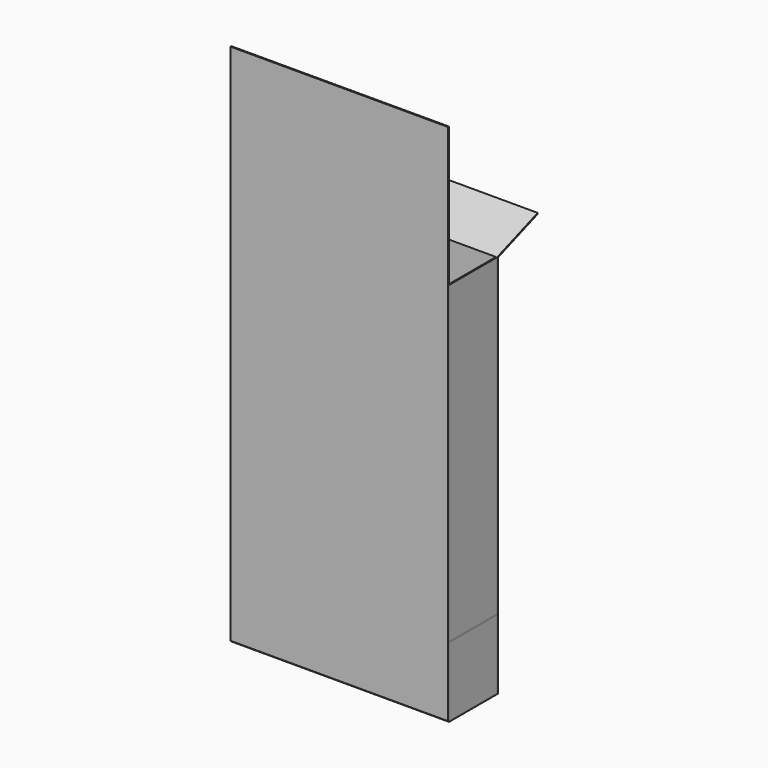
from build123d import *

# Parameters (mm, degrees)
F0_W      = 317.5
F0_H      = 762
F1_DEPTH  = 1.5875
F2_W      = 317.5
F2_H      = 88.9
F3_DEPTH  = 1.5875
F4_W      = 317.5
F4_H      = 558.8
F5_DEPTH  = 1.5875
F7_DEPTH  = 317.5
F8_DEPTH  = 1.5875
F11_DEPTH = 1.5875
F12_W     = 31.75
F12_H     = 78.7464009495
F13_DEPTH = 1.5875
F15_DEPTH = 2.54
F16_DEPTH = 1.5875
F6_W      = 87.3125
F6_H      = 1.5875
F17_DEPTH = 317.5
F6_H_2    = 100.0125
F18_DEPTH = 1.5875


# Not quite as in the source:
# - a length typed as a fraction of an inch, garbled in the dataset ("3 / 203.2 mm" for 3/8 in), is restored


with BuildPart() as f1:
    # F0 (on Front) → F1 (new body)
    with BuildSketch(Plane.XZ):
        Rectangle(F0_W, F0_H)
    extrude(amount=F1_DEPTH)


with BuildPart() as f3:
    # F2 (on face) → F3 (new body)
    with BuildSketch(Plane(origin=(0, 0, -381), x_dir=(1, 0, 0), z_dir=(0, 0, -1))):
        with Locations((0, -44.45)):
            Rectangle(F2_W, F2_H)
    extrude(amount=F3_DEPTH)

    # F4 (on face) → F5 (join)
    with BuildSketch(Plane(origin=(0, 88.9, 0), x_dir=(-1, 0, 0), z_dir=(0, 1, 0))):
        with Locations((0, -101.6)):
            Rectangle(F4_W, F4_H)
    extrude(amount=-F5_DEPTH)

    # F6 (on face) → F7 (join)
    with BuildSketch(Plane.YZ.offset(158.75)):
        Polygon((161.29, 204.7875), (87.3125, 177.8), (88.9, 177.8), (88.9, 176.7916309013), (161.29, 203.2), align=None)
    extrude(amount=-F7_DEPTH)

    # F12 (on face) → F13 (cut)
    with BuildSketch(Plane(origin=(0, -46.9892412703, 128.8058025409), x_dir=(1, 0, 0), z_dir=(0, -0.3427140755, 0.9394397599))):
        with Locations((15.875, 182.332597133)):
            Rectangle(F12_W, F12_H)
        with Locations((-15.875, 182.332597133)):
            Rectangle(F12_W, F12_H)
    extrude(amount=-F13_DEPTH, mode=Mode.SUBTRACT)

    # F15 (cut): a face of the model
    f15_faces = [f3.faces().sort_by_distance(p)[0] for p in [
        (0, 87.5845292974, 177.0543196906),
    ]]
    extrude(f15_faces, amount=-F15_DEPTH, mode=Mode.SUBTRACT)

    # F14 (on face) → F16 (cut)
    with BuildSketch(Plane(origin=(0, 88.9, 0), x_dir=(-1, 0, 0), z_dir=(0, 1, 0))):
        Polygon((31.75, 176.689293971), (0, 176.689293971), (-31.75, 176.689293971), (-31.75, -382.5875), (0, -382.5875), (31.75, -382.5875), align=None)
    extrude(amount=-F16_DEPTH, mode=Mode.SUBTRACT)


with BuildPart() as f8:
    # F6 (on face) → F8 (new body)
    with BuildSketch(Plane.YZ.offset(158.75)):
        Polygon((87.3125, 176.2125), (87.3125, 177.8), (0, 177.8), (0, -279.4), (87.3125, -279.4), align=None)
    extrude(amount=-F8_DEPTH)


with BuildPart() as f11:
    # F10 (on face) → F11 (new body)
    with BuildSketch(Plane(origin=(-158.75, 0, 0), x_dir=(0, -1, 0), z_dir=(-1, 0, 0))):
        Polygon((0, -381), (0, 177.8553873301), (-87.3104333878, 177.8553873301), (-87.3104333878, -381.0001015663), (0, -381.0001015663), align=None)
    extrude(amount=-F11_DEPTH)


with BuildPart() as f17:
    # F6 (on face) → F17 (new body)
    with BuildSketch(Plane.YZ.offset(158.75)):
        with Locations((43.65625, -280.19375)):
            Rectangle(F6_W, F6_H)
    extrude(amount=-F17_DEPTH)


with BuildPart() as f18:
    # F6 (on face) → F18 (new body)
    with BuildSketch(Plane.YZ.offset(158.75)):
        with Locations((43.65625, -330.99375)):
            Rectangle(F6_W, F6_H_2)
    extrude(amount=-F18_DEPTH)


solid = Compound([f1.part, f3.part, f8.part, f11.part, f17.part, f18.part])
